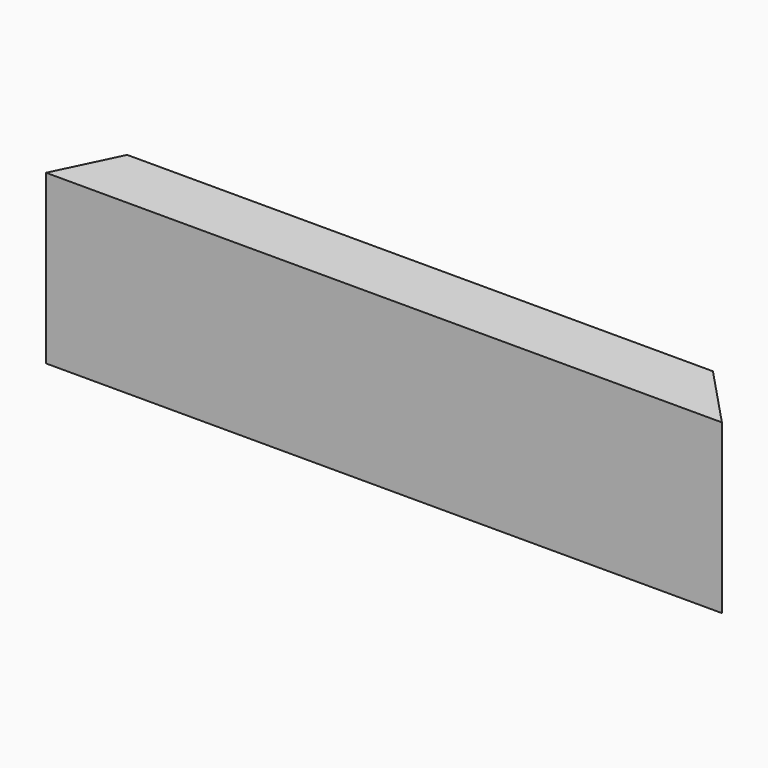
from build123d import *

# Parameters (mm, degrees)
F0_W     = 240
F0_H     = 59.62
F1_DEPTH = 16
F3_DEPTH = 240
F4_SIZE  = 15.99999


# Not quite as in the source:
# - a fillet or chamfer is up to 0.001 mm smaller than in the source, because OpenCascade refuses the exact size


with BuildPart() as f1:
    # F0 (on Front) → F1 (new body)
    with BuildSketch(Plane.XZ):
        with Locations((120, 29.81)):
            Rectangle(F0_W, F0_H)
    extrude(amount=F1_DEPTH)

    # F2 (on Right) → F3 (join)
    with BuildSketch(Plane.YZ):
        Polygon((0, 63.9071870789), (-16, 59.62), (0, 59.62), align=None)
    extrude(amount=F3_DEPTH)

    # F4 (size 16 in the source; OpenCascade refuses exactly that, so slightly less here)
    f4_edges = [f1.edges().sort_by_distance(p)[0] for p in [
        (0, 0, 31.953594),
        (120, 0, 0),
        (240, 0, 31.953594),
    ]]
    chamfer(f4_edges, length=F4_SIZE)


solid = f1.part
